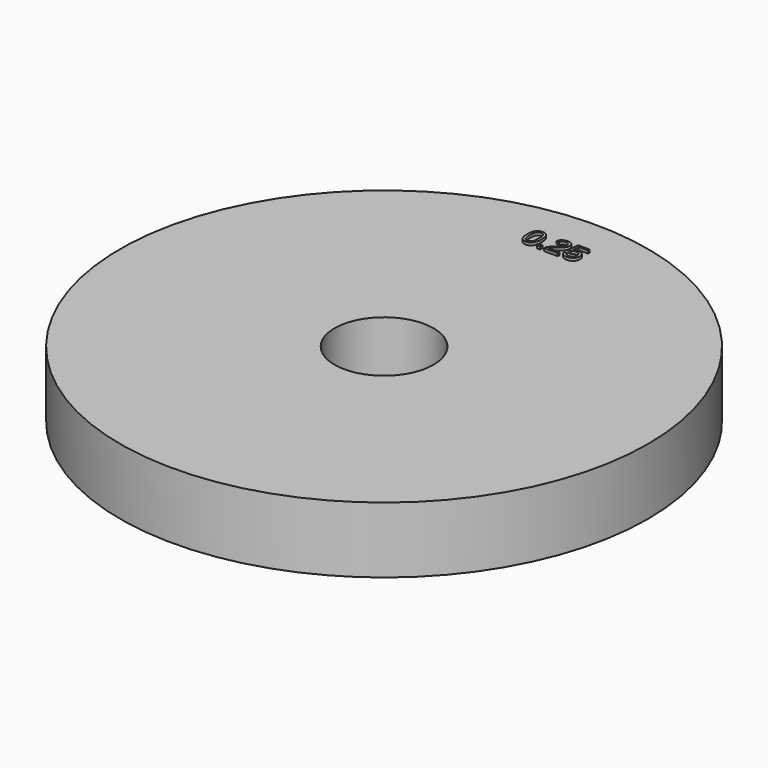
from build123d import *

# Parameters (mm, degrees)
F0_R         = 25.4
F0_R_2       = 4.7625
F1_DEPTH     = 6.35
F2_TEXT_SIZE = 2.8653817434
F3_DEPTH     = 0.254


# Not quite as in the source:
# - Text() gives the source's letters only with a copy of the font that has no kerning and outlines rounded to 1/6400 em; it was checked with that copy


with BuildPart() as f1:
    # F0 (on Top) → F1 (new body)
    with BuildSketch(Plane.XY):
        Circle(F0_R)
        Circle(F0_R_2, mode=Mode.SUBTRACT)
    extrude(amount=F1_DEPTH)

    # F2 (on face) → F3 (join)
    with BuildSketch(Plane.XY.offset(6.35)):
        with Locations((-2.8275497501, 19.6224143729)):
            Text('0.25', F2_TEXT_SIZE, font='Arimo', text_align=(TextAlign.LEFT, TextAlign.BOTTOM))
    extrude(amount=F3_DEPTH)


solid = f1.part
